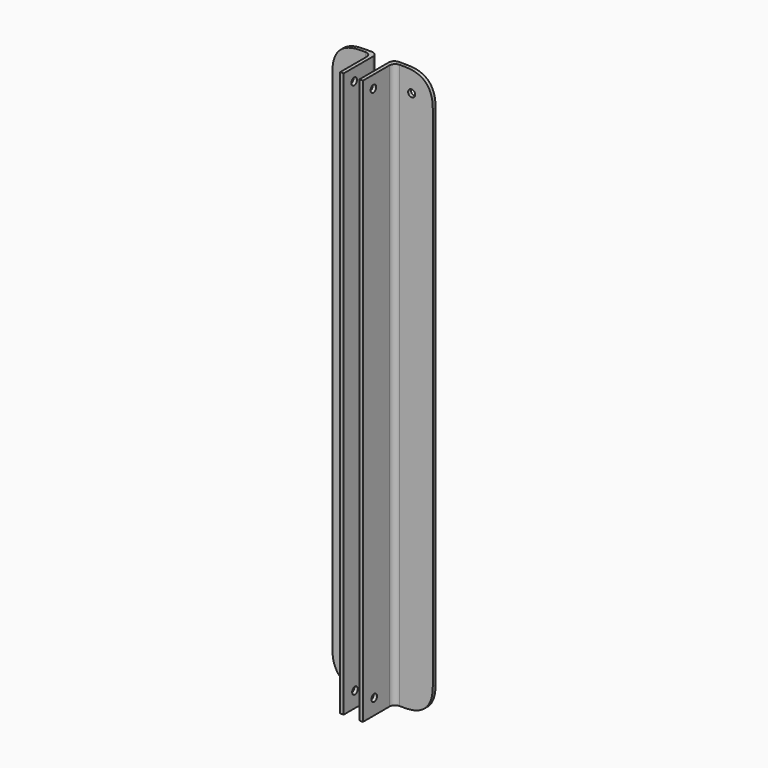
from build123d import *

# Parameters (mm, degrees)
F1_DEPTH       = 508
F2_R           = 3.175
F3_DEPTH       = 3.175
F4_R           = 3.175
F5_DEPTH       = 3.175
F7_DEPTH       = 508
F8_R           = 3.175
F9_DEPTH       = 3.175
F10_R          = 3.175
F11_DEPTH      = 3.175
F12_R          = 3.175
F13_DEPTH      = 3.175
F14_T1_DEPTH   = 130.175
F16_T1_DEPTH   = 130.175
F15_R          = 3.175
F17_DEPTH      = 3.175
F18_T1_DEPTH   = 130.175
F18_2_T1_DEPTH = 130.175
F19_R          = 5.08
F19_2_R        = 5.08


# Not quite as in the source:
# - a fillet or chamfer that OpenCascade refuses, or shapes differently, is made with other operations: its cross-section is extruded or revolved along the edge and cut away or added


with BuildPart() as f1:
    # F0 (on Top) → F1 (new body)
    with BuildSketch(Plane.XY):
        Polygon((-34.925, 24.1499475421), (-34.925, 20.9749475421), (0, 20.9749475421), (0, -13.9500524579), (3.175, -13.9500524579), (3.175, 24.1499475421), align=None)
    extrude(amount=F1_DEPTH)

    # F2 (on face) → F3 (cut)
    with BuildSketch(Plane(origin=(0, 0, 0), x_dir=(0, -1, 0), z_dir=(-1, 0, 0))):
        with Locations((2.1390524579, 496.824)):
            Circle(F2_R)
    extrude(amount=-F3_DEPTH, mode=Mode.SUBTRACT)

    # F4 (on face) → F5 (cut)
    with BuildSketch(Plane(origin=(0, 0, 0), x_dir=(0, -1, 0), z_dir=(-1, 0, 0))):
        with Locations((1.2500524579, 13.97)):
            Circle(F4_R)
    extrude(amount=-F5_DEPTH, mode=Mode.SUBTRACT)

    # F16: fillet of radius 25.4 on 1 edges, made by hand

    # F16_s2 → F16_t1 (cut)
    with BuildSketch(Plane.XZ.offset(-87.6499475421)):
        with BuildLine():
            add(Edge.make_bspline(
                [(-34.925, 482.6), (-34.925, 508), (-9.525, 508)],
                knots=[0, 0, 0, 1, 1, 1], degree=2, weights=[1, 1, 1]))
            Line((-9.525, 508), (-34.925, 508))
            Line((-34.925, 508), (-34.925, 482.6))
        make_face()
    extrude(amount=F16_T1_DEPTH, mode=Mode.SUBTRACT)

    # F15 (on face) → F17 (cut)
    with BuildSketch(Plane(origin=(0, 24.1499475421, 0), x_dir=(-1, 0, 0), z_dir=(0, 1, 0))):
        with Locations((15.875, 488.95)):
            Circle(F15_R)
    extrude(amount=-F17_DEPTH, mode=Mode.SUBTRACT)

    # F18#2: fillet of radius 25.4 on 1 edges, made by hand

    # F18_2_s2 → F18_2_t1 (cut)
    with BuildSketch(Plane.XZ.offset(-87.6499475421)):
        with BuildLine():
            add(Edge.make_bspline(
                [(-9.525, 0), (-34.925, 0), (-34.925, 25.4)],
                knots=[0, 0, 0, 1, 1, 1], degree=2, weights=[1, 1, 1]))
            Line((-34.925, 25.4), (-34.925, 0))
            Line((-34.925, 0), (-9.525, 0))
        make_face()
    extrude(amount=F18_2_T1_DEPTH, mode=Mode.SUBTRACT)

    # F19#2
    f19_2_edges = [f1.edges().sort_by_distance(p)[0] for p in [
        (0, 20.974948, 254),
        (3.175, 24.149948, 254),
    ]]
    fillet(f19_2_edges, radius=F19_2_R)


with BuildPart() as f7:
    # F6 (on Top) → F7 (new body)
    with BuildSketch(Plane.XY):
        Polygon((17.4523038154, 23.9860548146), (17.4523038154, -14.1139451854), (20.6273038154, -14.1139451854), (20.6273038154, 20.8110548146), (55.5523038154, 20.8110548146), (55.5523038154, 23.9860548146), align=None)
    extrude(amount=F7_DEPTH)

    # F8 (on face) → F9 (cut)
    with BuildSketch(Plane(origin=(17.4523038154, 0, 0), x_dir=(0, -1, 0), z_dir=(-1, 0, 0))):
        with Locations((2.3029451854, 496.824)):
            Circle(F8_R)
    extrude(amount=-F9_DEPTH, mode=Mode.SUBTRACT)

    # F10 (on face) → F11 (cut)
    with BuildSketch(Plane(origin=(17.4523038154, 0, 0), x_dir=(0, -1, 0), z_dir=(-1, 0, 0))):
        with Locations((1.4139451854, 13.97)):
            Circle(F10_R)
    extrude(amount=-F11_DEPTH, mode=Mode.SUBTRACT)

    # F12 (on face) → F13 (cut)
    with BuildSketch(Plane(origin=(0, 23.9860548146, 0), x_dir=(-1, 0, 0), z_dir=(0, 1, 0))):
        with Locations((-36.5023038154, 488.95)):
            Circle(F12_R)
    extrude(amount=-F13_DEPTH, mode=Mode.SUBTRACT)

    # F14: fillet of radius 25.4 on 1 edges, made by hand

    # F14_s2 → F14_t1 (cut)
    with BuildSketch(Plane.XZ.offset(-87.4860548146)):
        with BuildLine():
            add(Edge.make_bspline(
                [(55.5523038154, 482.6), (55.5523038154, 508), (30.1523038154, 508)],
                knots=[0, 0, 0, 1, 1, 1], degree=2, weights=[1, 1, 1]))
            Line((30.1523038154, 508), (55.5523038154, 508))
            Line((55.5523038154, 508), (55.5523038154, 482.6))
        make_face()
    extrude(amount=F14_T1_DEPTH, mode=Mode.SUBTRACT)

    # F18: fillet of radius 25.4 on 1 edges, made by hand

    # F18_s2 → F18_t1 (cut)
    with BuildSketch(Plane.XZ.offset(-87.4860548146)):
        with BuildLine():
            add(Edge.make_bspline(
                [(30.1523038154, 0), (55.5523038154, 0), (55.5523038154, 25.4)],
                knots=[0, 0, 0, 1, 1, 1], degree=2, weights=[1, 1, 1]))
            Line((55.5523038154, 25.4), (55.5523038154, 0))
            Line((55.5523038154, 0), (30.1523038154, 0))
        make_face()
    extrude(amount=F18_T1_DEPTH, mode=Mode.SUBTRACT)

    # F19
    f19_edges = [f7.edges().sort_by_distance(p)[0] for p in [
        (20.627304, 20.811055, 254),
        (17.452304, 23.986055, 254),
    ]]
    fillet(f19_edges, radius=F19_R)


solid = Compound([f1.part, f7.part])
